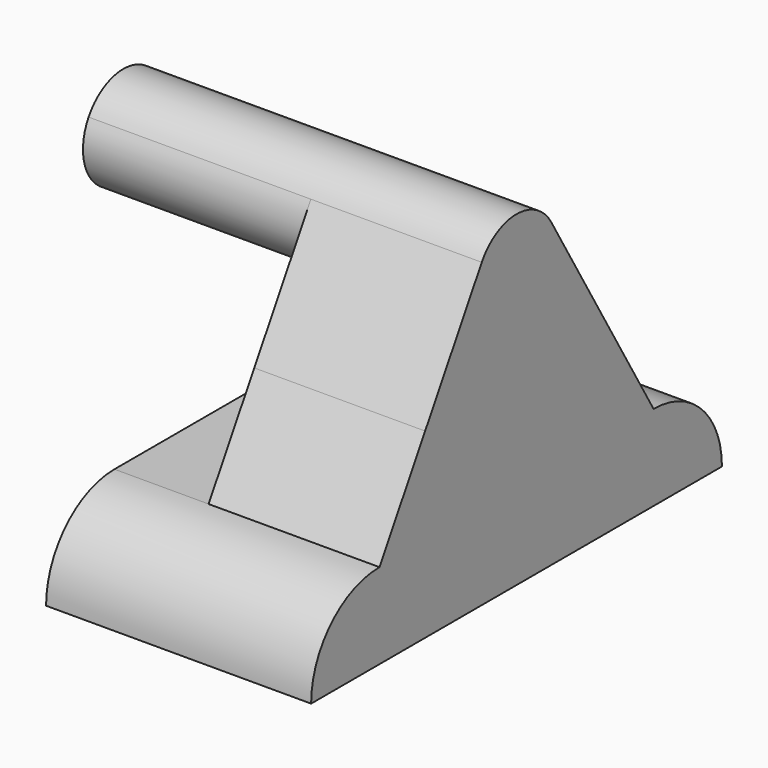
from build123d import *

# Parameters (mm, degrees)
F0_W           = 8.4991231561
F0_H           = 6.35
F1_DEPTH       = 12.7
F2_DEPTH       = 16.525
F3_DEPTH       = 7
F5_D           = 3.4544
F5_DEPTH       = 12.7
F5_CSINK_D     = 4.5974
F5_CSINK_ANGLE = 82
F5_TIP         = 1.0378064612


# Not quite as in the source:
# - a length typed as a fraction of an inch, garbled in the dataset ("3 / 203.2 mm" for 3/8 in), is restored


with BuildPart() as f1:
    # F0 (on Right) → F1 (new body)
    with BuildSketch(Plane.YZ):
        with BuildLine():
            ThreePointArc((19.0844833851, -6.525), (17.2246114456, -2.0348719395), (12.7344833851, -0.175))
            Line((12.7344833851, -0.175), (8.4991231561, -0.175))
            Line((8.4991231561, -0.175), (8.4991231561, -6.525))
            Line((8.4991231561, -6.525), (19.0844833851, -6.525))
        make_face()
        with BuildLine():
            Line((-8.4991231561, -0.175), (-12.7344833851, -0.175))
            ThreePointArc((-12.7344833851, -0.175), (-17.2246114456, -2.0348719395), (-19.0844833851, -6.525))
            Line((-19.0844833851, -6.525), (-8.4991231561, -6.525))
            Line((-8.4991231561, -6.525), (-8.4991231561, -0.175))
        make_face()
        with BuildLine():
            ThreePointArc((8.4901041675, 7.0058502143), (0, 3), (-8.4901041675, 7.0058502143))
            Line((-8.4901041675, 7.0058502143), (-12.7344833851, -0.175))
            Line((-12.7344833851, -0.175), (-8.4991231561, -0.175))
            Line((-8.4991231561, -0.175), (0, -0.175))
            Line((0, -0.175), (8.4991231561, -0.175))
            Line((8.4991231561, -0.175), (12.7344833851, -0.175))
            Line((12.7344833851, -0.175), (8.4901041675, 7.0058502143))
        make_face()
        with BuildLine():
            Line((-3.2282481135, 15.9081179517), (-8.4901041675, 7.0058502143))
            ThreePointArc((-8.4901041675, 7.0058502143), (0, 3), (8.4901041675, 7.0058502143))
            Line((8.4901041675, 7.0058502143), (3.2282481135, 15.9081179517))
            ThreePointArc((3.2282481135, 15.9081179517), (3.6172109716, 14.9890828009), (3.75, 14))
            ThreePointArc((3.75, 14), (-0.9890828009, 10.3827890284), (-3.2282481135, 15.9081179517))
        make_face()
        with BuildLine():
            ThreePointArc((3.2282481135, 15.9081179517), (0, 17.75), (-3.2282481135, 15.9081179517))
            ThreePointArc((-3.2282481135, 15.9081179517), (-0.9890828009, 10.3827890284), (3.75, 14))
            ThreePointArc((3.75, 14), (3.6172109716, 14.9890828009), (3.2282481135, 15.9081179517))
        make_face()
        with Locations((4.249561578, -3.35)):
            Rectangle(F0_W, F0_H)
        with Locations((-4.249561578, -3.35)):
            Rectangle(F0_W, F0_H)
    extrude(amount=F1_DEPTH)

    # F0 (on Right) → F2 (join)
    with BuildSketch(Plane.YZ):
        with BuildLine():
            ThreePointArc((3.2282481135, 15.9081179517), (0, 17.75), (-3.2282481135, 15.9081179517))
            ThreePointArc((-3.2282481135, 15.9081179517), (-0.9890828009, 10.3827890284), (3.75, 14))
            ThreePointArc((3.75, 14), (3.6172109716, 14.9890828009), (3.2282481135, 15.9081179517))
        make_face()
    extrude(amount=-F2_DEPTH)

    # F0 (on Right) → F3 (join)
    with BuildSketch(Plane.YZ):
        with BuildLine():
            ThreePointArc((19.0844833851, -6.525), (17.2246114456, -2.0348719395), (12.7344833851, -0.175))
            Line((12.7344833851, -0.175), (8.4991231561, -0.175))
            Line((8.4991231561, -0.175), (8.4991231561, -6.525))
            Line((8.4991231561, -6.525), (19.0844833851, -6.525))
        make_face()
        with BuildLine():
            Line((-8.4991231561, -0.175), (-12.7344833851, -0.175))
            ThreePointArc((-12.7344833851, -0.175), (-17.2246114456, -2.0348719395), (-19.0844833851, -6.525))
            Line((-19.0844833851, -6.525), (-8.4991231561, -6.525))
            Line((-8.4991231561, -6.525), (-8.4991231561, -0.175))
        make_face()
        with Locations((4.249561578, -3.35)):
            Rectangle(F0_W, F0_H)
        with Locations((-4.249561578, -3.35)):
            Rectangle(F0_W, F0_H)
    extrude(amount=-F3_DEPTH)

    # F5
    with Locations(Plane(origin=(0, 0, -6.525), x_dir=(1, 0, 0), z_dir=(0, 0, -1))):
        with Locations((6.35, 0)):
            CounterSinkHole(F5_D / 2, F5_CSINK_D / 2, depth=F5_DEPTH, counter_sink_angle=F5_CSINK_ANGLE)
            with Locations((0, 0, -(F5_DEPTH + F5_TIP / 2))):  # 118° drill point
                Cone(0, F5_D / 2, F5_TIP, mode=Mode.SUBTRACT)


solid = f1.part
